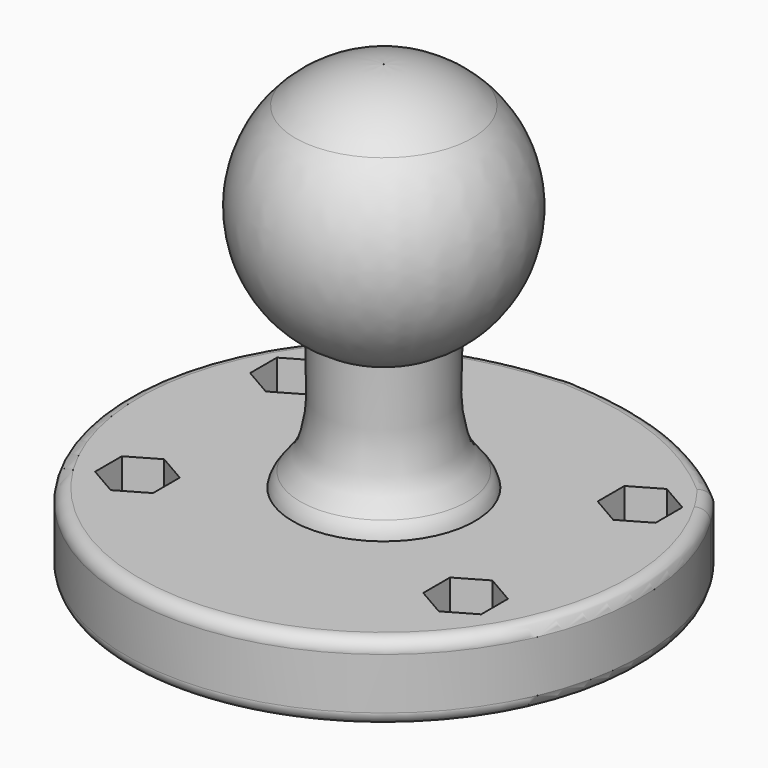
from build123d import *

# Parameters (mm, degrees)
F0_R     = 2.5
F1_DEPTH = 12
F3_R     = 2.5
F4_DEPTH = 6
F5_R     = 2


# Not quite as in the source:
# - a fillet or chamfer that OpenCascade refuses, or shapes differently, is made with other operations: its cross-section is extruded or revolved along the edge and cut away or added


with BuildPart() as f1:
    # F0 (on Top) → F1 (new body)
    with BuildSketch(Plane.XY):
        with BuildLine():
            ThreePointArc((-31.3651592039, 24.7400687451), (-33.0304528025, 22.4689333996), (-34.5318159842, 20.0862527403))
            ThreePointArc((-34.5318159842, 20.0862527403), (0.3556410553, -40.0322385106), (34.289361103, 20.6296959515))
            ThreePointArc((34.289361103, 20.6296959515), (32.9313235996, 22.7293613836), (31.4447447441, 24.7400687451))
            add(Edge.make_bspline(
                [(31.4447447441, 24.7400687451), (22.988602022, 32.1085255021), (13.1297165658, 36.2919575894), (0.0397927701, 36.9132596428)],
                knots=[0, 0, 0, 0, 0.5, 0.5, 0.5, 0.5], degree=3))
            add(Edge.make_bspline(
                [(-31.3651592039, 24.7400687451), (-22.9090164817, 32.1085255021), (-13.0501310255, 36.2919575894), (0.0397927701, 36.9132596428)],
                knots=[0, 0, 0, 0, 0.5, 0.5, 0.5, 0.5], degree=3))
        make_face()
        with Locations((-25.4602072299, -16.0334855318)):
            Circle(F0_R, mode=Mode.SUBTRACT)
        with Locations((25.5397927701, -16.0334855318)):
            Circle(F0_R, mode=Mode.SUBTRACT)
        with Locations((-26.9602072299, 15.9665144682)):
            Circle(F0_R, mode=Mode.SUBTRACT)
        with Locations((27.0397927701, 15.9665144682)):
            Circle(F0_R, mode=Mode.SUBTRACT)
    extrude(amount=F1_DEPTH)

    # F3 (on face) → F4 (cut)
    with BuildSketch(Plane.XY.offset(12)):
        Polygon((-22.4602072299, 13.3684382568), (-22.4602072299, 18.5645906795), (-26.9602072299, 21.1626668909), (-31.4602072299, 18.5645906795), (-31.4602072299, 13.3684382568), (-26.9602072299, 10.7703620455), align=None)
        with Locations((-26.9602072299, 15.9665144682)):
            Circle(F3_R, mode=Mode.SUBTRACT)
        Polygon((22.5397927701, 18.5645906795), (22.5397927701, 13.3684382568), (27.0397927701, 10.7703620455), (31.5397927701, 13.3684382568), (31.5397927701, 18.5645906795), (27.0397927701, 21.1626668909), align=None)
        with Locations((27.0397927701, 15.9665144682)):
            Circle(F3_R, mode=Mode.SUBTRACT)
        Polygon((21.0397927701, -13.4354093205), (21.0397927701, -18.6315617432), (25.5397927701, -21.2296379545), (30.0397927701, -18.6315617432), (30.0397927701, -13.4354093205), (25.5397927701, -10.8373331091), align=None)
        with Locations((25.5397927701, -16.0334855318)):
            Circle(F3_R, mode=Mode.SUBTRACT)
        Polygon((-20.9602072299, -18.6315617432), (-20.9602072299, -13.4354093205), (-25.4602072299, -10.8373331091), (-29.9602072299, -13.4354093205), (-29.9602072299, -18.6315617432), (-25.4602072299, -21.2296379545), align=None)
        with Locations((-25.4602072299, -16.0334855318)):
            Circle(F3_R, mode=Mode.SUBTRACT)
    extrude(amount=-F4_DEPTH, mode=Mode.SUBTRACT)

    # F5
    f5_edges = [f1.edges().sort_by_distance(p)[0] for p in [
        (-2.459557, -39.955325, 12),
        (-2.459557, -39.955325, 0),
        (16.831403, 33.608309, 12),
        (-16.751817, 33.608309, 12),
        (-16.751817, 33.608309, 0),
        (16.831403, 33.608309, 0),
    ]]
    fillet(f5_edges, radius=F5_R)

    # F6 (on Front) → F7 (revolve)
    with BuildSketch(Plane.XZ):
        with BuildLine():
            Line((-14.1540115437, 11.8460487906), (-0.0248217459, 11.8460487906))
            Line((-0.0248217459, 11.8460487906), (-0.0248217459, 12.5021283307))
            Line((-0.0248217459, 12.5021283307), (-0.0248217459, 25.1048319042))
            Line((-0.0248217459, 25.1048319042), (-0.0248217459, 58.8260033315))
            Line((-0.0248217459, 58.8260033315), (-0.0248217459, 64.264058532))
            Line((-0.0248217459, 64.264058532), (-0.0248217459, 69.9135838276))
            ThreePointArc((-0.0248217459, 69.9135838276), (-7.4432934465, 68.4459215755), (-13.744069299, 64.264058532))
            ThreePointArc((-13.744069299, 64.264058532), (-19.3321206406, 47.8233148814), (-9.582830593, 33.4540520906))
            add(Edge.make_bspline(
                [(-14.1540115437, 13.0516188551), (-12.6789047108, 14.5682779679), (-8.9868889419, 18.3642941178), (-9.359245349, 27.7926803584), (-9.582830593, 33.4540520906)],
                knots=[0, 0, 0, 0, 0.3995396892, 1, 1, 1, 1], degree=3))
            Line((-14.1540115437, 13.0516188551), (-14.1540115437, 11.8460487906))
        make_face()
    revolve(axis=Axis((0, 0, 50.5361706018), (0, 0, 1)))

    # F8: fillet of radius 5 on 1 edges, made by hand

    # F8_s1 → F8_t2 (revolve, cut)
    with BuildSketch(Plane.XZ):
        with BuildLine():
            ThreePointArc((-14.1540115437, 12), (-13.716188898, 13.2222804174), (-12.9784286022, 14.2906285974))
            Line((-12.9784286022, 14.2906285974), (-13.0526409195, 14.3576549502))
            ThreePointArc((-13.0526409195, 14.3576549502), (-13.6328295807, 13.7347113697), (-14.2256974002, 13.1213407167))
            Line((-14.2256974002, 13.1213407167), (-14.2540115437, 13.0516188551))
            ThreePointArc((-14.2540115437, 13.0516188551), (-14.2540115437, 12.5258094276), (-14.2517355198, 12.0212137808))
            Line((-14.2517355198, 12.0212137808), (-14.1540115437, 12))
        make_face()
    revolve(axis=Axis((0, 0, 13.0516188551), (0, 0, 1)), mode=Mode.SUBTRACT)


solid = f1.part
